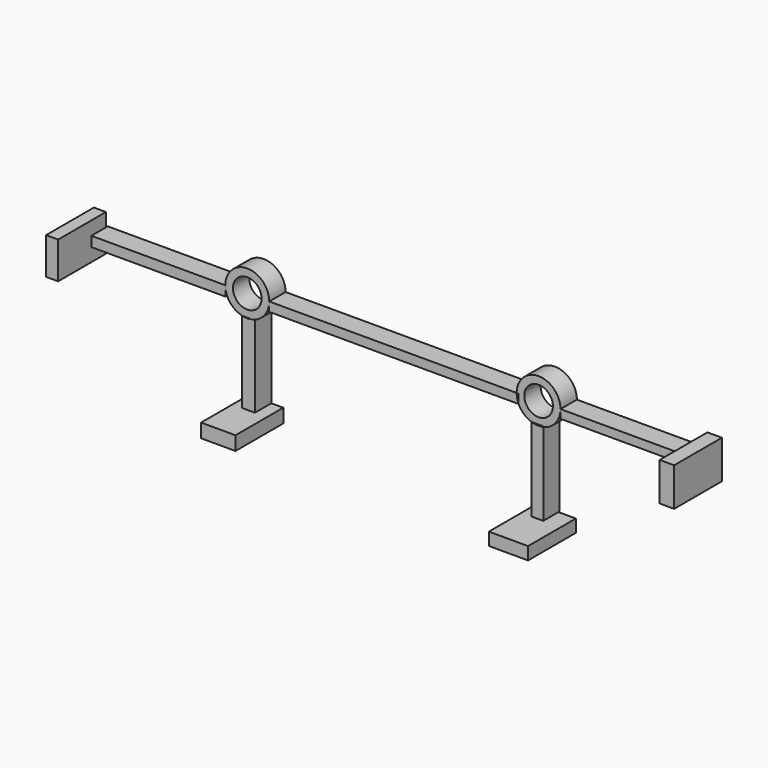
from build123d import *

# Parameters (mm, degrees)
F0_W     = 19.6500662714
F0_H     = 1.2726495042
F1_DEPTH = 3.048
F0_R     = 2.1336
F0_R_2   = 2.1294315388
F0_W_2   = 19.939
F0_H_2   = 1.4862371609
F2_W     = 1.7960518599
F2_H     = 5.4779564962
F3_DEPTH = 8.89
F2_W_2   = 5.1187463105
F2_H_2   = 2.0654590335
F2_W_3   = 5.8371666819
F2_H_3   = 1.8858539406
F2_W_4   = 2.1589994431
F2_H_4   = 5.7150004432


with BuildPart() as f1:
    # F0 (on Front) → F1 (new body)
    with BuildSketch(Plane.XZ):
        with Locations((31.9208344445, 12.1880299412)):
            Rectangle(F0_W, F0_H)
    extrude(amount=F1_DEPTH)


with BuildPart() as f1b:
    # F0 (on Front) → F1, piece 2 (new body)
    with BuildSketch(Plane.XZ):
        with BuildLine():
            ThreePointArc((22.0958013088, 12.8243546933), (18.8319013088, 16.0882546933), (15.5680013088, 12.8243546933))
            Line((15.5680013088, 12.8243546933), (15.8661592174, 12.8243546933))
            Line((15.8661592174, 12.8243546933), (15.8661592174, 11.4614838053))
            ThreePointArc((15.8661592174, 11.4614838053), (16.6448945696, 10.4015371738), (17.778771361, 9.7350245842))
            Line((17.778771361, 9.7350245842), (19.5327494293, 9.7350245842))
            Line((19.5327494293, 9.7350245842), (19.5327494293, 9.6365882147))
            ThreePointArc((19.5327494293, 9.6365882147), (21.3755739873, 10.7791719351), (22.0958013088, 12.8243546933))
        make_face()
        with Locations((18.8319013088, 12.8243546933)):
            Circle(F0_R, mode=Mode.SUBTRACT)
    extrude(amount=F1_DEPTH)


with BuildPart() as f1c:
    # F0 (on Front) → F1, piece 3 (new body)
    with BuildSketch(Plane.XZ):
        with BuildLine():
            Line((15.5680013088, 12.8243546933), (-21.2678752836, 12.8243546933))
            Line((-21.2678752836, 12.8243546933), (-21.2678752836, 11.4614838053))
            Line((-21.2678752836, 11.4614838053), (15.8661592174, 11.4614838053))
            ThreePointArc((15.8661592174, 11.4614838053), (15.6434119468, 12.1268026888), (15.5680013088, 12.8243546933))
        make_face()
    extrude(amount=F1_DEPTH)


with BuildPart() as f1d:
    # F0 (on Front) → F1, piece 4 (new body)
    with BuildSketch(Plane.XZ):
        with BuildLine():
            ThreePointArc((-23.7866874056, 9.6416087265), (-21.9737613738, 10.7949282722), (-21.2678752836, 12.8243546933))
            ThreePointArc((-21.2678752836, 12.8243546933), (-24.5381244323, 16.0946038419), (-27.8083735809, 12.8243546933))
            ThreePointArc((-27.8083735809, 12.8243546933), (-27.1024874907, 10.7949282722), (-25.2895614589, 9.6416087265))
            Line((-25.2895614589, 9.6416087265), (-23.7866874056, 9.6416087265))
        make_face()
        with Locations((-24.5381244323, 12.8243546933)):
            Circle(F0_R_2, mode=Mode.SUBTRACT)
    extrude(amount=F1_DEPTH)


with BuildPart() as f1e:
    # F0 (on Front) → F1, piece 5 (new body)
    with BuildSketch(Plane.XZ):
        with Locations((-37.7778735809, 12.0812361129)):
            Rectangle(F0_W_2, F0_H_2)
    extrude(amount=F1_DEPTH)


with BuildPart() as f1f:
    # F0 (on Front) → F1, piece 6 (new body)
    with BuildSketch(Plane.XZ):
        with BuildLine():
            Line((-23.3983788639, 9.6416087265), (-23.7866874056, 9.6416087265))
            ThreePointArc((-23.7866874056, 9.6416087265), (-24.5381244323, 9.5541055446), (-25.2895614589, 9.6416087265))
            Line((-25.2895614589, 9.6416087265), (-25.2895614589, -2.7586696669))
            Line((-25.2895614589, -2.7586696669), (-23.3983788639, -2.7586696669))
            Line((-23.3983788639, -2.7586696669), (-23.3983788639, 9.6416087265))
        make_face()
    extrude(amount=F1_DEPTH)


with BuildPart() as f1g:
    # F0 (on Front) → F1, piece 7 (new body)
    with BuildSketch(Plane.XZ):
        with BuildLine():
            Line((19.5327494293, -2.6601754158), (19.5327494293, 9.6365882147))
            ThreePointArc((19.5327494293, 9.6365882147), (18.6490132251, 9.5655826609), (17.778771361, 9.7350245842))
            Line((17.778771361, 9.7350245842), (17.778771361, -2.6601754158))
            Line((17.778771361, -2.6601754158), (19.5327494293, -2.6601754158))
        make_face()
    extrude(amount=F1_DEPTH)


with BuildPart() as f3:
    # F2 (on Front) → F3 (new body)
    with BuildSketch(Plane.XZ):
        with Locations((-48.9171035588, 11.8750003166)):
            Rectangle(F2_W, F2_H)
    extrude(amount=F3_DEPTH)


with BuildPart() as f3b:
    # F2 (on Front) → F3, piece 2 (new body)
    with BuildSketch(Plane.XZ):
        with Locations((-24.1764970124, -3.4812387312)):
            Rectangle(F2_W_2, F2_H_2)
    extrude(amount=F3_DEPTH)


with BuildPart() as f3c:
    # F2 (on Front) → F3, piece 3 (new body)
    with BuildSketch(Plane.XZ):
        with Locations((19.0185336396, -3.7506463705)):
            Rectangle(F2_W_3, F2_H_3)
    extrude(amount=F3_DEPTH)


with BuildPart() as f3d:
    # F2 (on Front) → F3, piece 4 (new body)
    with BuildSketch(Plane.XZ):
        with Locations((42.608499527, 11.9988550432)):
            Rectangle(F2_W_4, F2_H_4)
    extrude(amount=F3_DEPTH)


solid = Compound([f1.part, f1b.part, f1c.part, f1d.part, f1e.part, f1f.part, f1g.part, f3.part, f3b.part, f3c.part, f3d.part])
